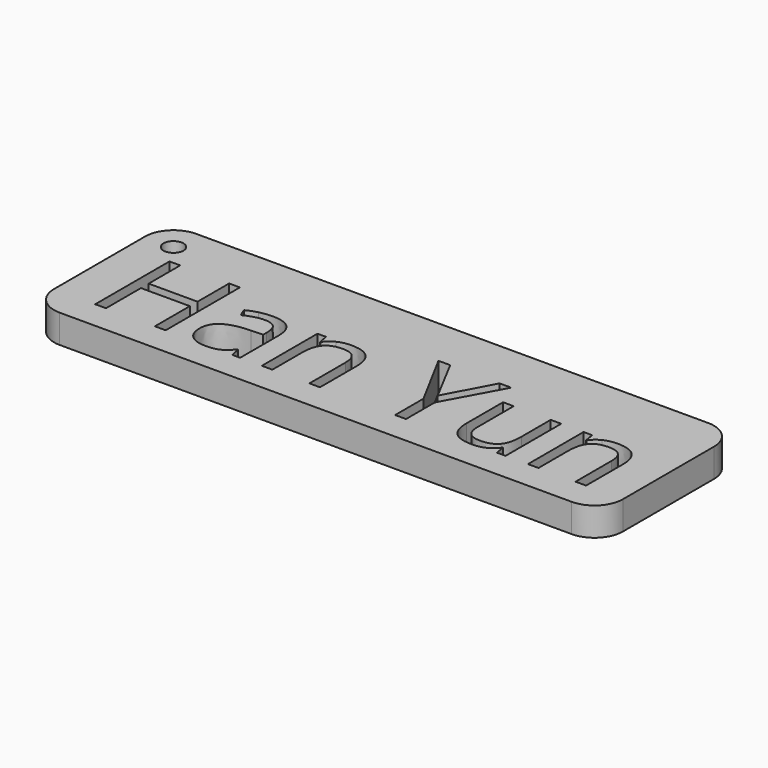
from build123d import *

# Parameters (mm, degrees)
F0_R     = 1.75
F1_DEPTH = 5


with BuildPart() as f1:
    # F0 (on Top) → F1 (new body)
    with BuildSketch(Plane.XY):
        with BuildLine():
            Line((95, 0), (5, 0))
            ThreePointArc((5, 0), (1.4644660941, -1.4644660941), (0, -5))
            Line((0, -5), (0, -25))
            ThreePointArc((0, -25), (1.4644660941, -28.5355339059), (5, -30))
            Line((5, -30), (95, -30))
            ThreePointArc((95, -30), (98.5355339059, -28.5355339059), (100, -25))
            Line((100, -25), (100, -5))
            ThreePointArc((100, -5), (98.5355339059, -1.4644660941), (95, 0))
        make_face()
        Polygon((19.6251784864, -8.6899095669), (19.6251784864, -25), (17.7296525464, -25), (17.7296525464, -17.3250832937), (9.137315564, -17.3250832937), (9.137315564, -25), (7.241789624, -25), (7.241789624, -8.6899095669), (9.137315564, -8.6899095669), (9.137315564, -15.6294621609), (17.7296525464, -15.6294621609), (17.7296525464, -8.6899095669), align=None, mode=Mode.SUBTRACT)
        with BuildLine():
            Line((32.7118039029, -25), (31.3374583532, -25))
            Line((31.3374583532, -25), (30.969776297, -23.2579723941))
            Line((30.969776297, -23.2579723941), (30.8805330795, -23.2579723941))
            add(Edge.make_bspline(
                [(30.8805330795, -23.2579723941), (29.9666825321, -24.4074250357), (29.0581865778, -24.8161589719)],
                knots=[0, 0, 0, 1, 1, 1], degree=2))
            add(Edge.make_bspline(
                [(29.0581865778, -24.8161589719), (28.1496906235, -25.2248929081), (26.7860542599, -25.2248929081)],
                knots=[0, 0, 0, 1, 1, 1], degree=2))
            add(Edge.make_bspline(
                [(26.7860542599, -25.2248929081), (24.9690623513, -25.2248929081), (23.9374107568, -24.2860542599)],
                knots=[0, 0, 0, 1, 1, 1], degree=2))
            add(Edge.make_bspline(
                [(23.9374107568, -24.2860542599), (22.9057591623, -23.3472156116), (22.9057591623, -21.6194669205)],
                knots=[0, 0, 0, 1, 1, 1], degree=2))
            add(Edge.make_bspline(
                [(22.9057591623, -21.6194669205), (22.9057591623, -17.917658258), (28.8279390766, -17.7391718229)],
                knots=[0, 0, 0, 1, 1, 1], degree=2))
            Line((28.8279390766, -17.7391718229), (30.9019514517, -17.6713469776))
            Line((30.9019514517, -17.6713469776), (30.9019514517, -16.9109947644))
            add(Edge.make_bspline(
                [(30.9019514517, -16.9109947644), (30.9019514517, -15.472394098), (30.2843883865, -14.7870061875)],
                knots=[0, 0, 0, 1, 1, 1], degree=2))
            add(Edge.make_bspline(
                [(30.2843883865, -14.7870061875), (29.6668253213, -14.101618277), (28.3031889576, -14.101618277)],
                knots=[0, 0, 0, 1, 1, 1], degree=2))
            add(Edge.make_bspline(
                [(28.3031889576, -14.101618277), (26.7753450738, -14.101618277), (24.8476915754, -15.0368871966)],
                knots=[0, 0, 0, 1, 1, 1], degree=2))
            Line((24.8476915754, -15.0368871966), (24.2765349833, -13.6197049024))
            add(Edge.make_bspline(
                [(24.2765349833, -13.6197049024), (25.1796763446, -13.1306520704), (26.2559495478, -12.8522132318)],
                knots=[0, 0, 0, 1, 1, 1], degree=2))
            add(Edge.make_bspline(
                [(26.2559495478, -12.8522132318), (27.3322227511, -12.5737743931), (28.4174202761, -12.5737743931)],
                knots=[0, 0, 0, 1, 1, 1], degree=2))
            add(Edge.make_bspline(
                [(28.4174202761, -12.5737743931), (30.6020942408, -12.5737743931), (31.6569490719, -13.5429557354)],
                knots=[0, 0, 0, 1, 1, 1], degree=2))
            add(Edge.make_bspline(
                [(31.6569490719, -13.5429557354), (32.7118039029, -14.5121370776), (32.7118039029, -16.653974298)],
                knots=[0, 0, 0, 1, 1, 1], degree=2))
            Line((32.7118039029, -16.653974298), (32.7118039029, -25))
        make_face(mode=Mode.SUBTRACT)
        with BuildLine():
            Line((46.744407425, -25), (44.8917182294, -25))
            Line((44.8917182294, -25), (44.8917182294, -17.0894811994))
            add(Edge.make_bspline(
                [(44.8917182294, -17.0894811994), (44.8917182294, -15.5973346026), (44.2116849119, -14.8601856259)],
                knots=[0, 0, 0, 1, 1, 1], degree=2))
            add(Edge.make_bspline(
                [(44.2116849119, -14.8601856259), (43.5316515945, -14.1230366492), (42.0787720133, -14.1230366492)],
                knots=[0, 0, 0, 1, 1, 1], degree=2))
            add(Edge.make_bspline(
                [(42.0787720133, -14.1230366492), (40.1618277011, -14.1230366492), (39.2693955259, -15.1600428367)],
                knots=[0, 0, 0, 1, 1, 1], degree=2))
            add(Edge.make_bspline(
                [(39.2693955259, -15.1600428367), (38.3769633508, -16.1970490243), (38.3769633508, -18.585197525)],
                knots=[0, 0, 0, 1, 1, 1], degree=2))
            Line((38.3769633508, -18.585197525), (38.3769633508, -25))
            Line((38.3769633508, -25), (36.5242741552, -25))
            Line((36.5242741552, -25), (36.5242741552, -12.7736792004))
            Line((36.5242741552, -12.7736792004), (38.0306996668, -12.7736792004))
            Line((38.0306996668, -12.7736792004), (38.3305568777, -14.447881961))
            Line((38.3305568777, -14.447881961), (38.4198000952, -14.447881961))
            add(Edge.make_bspline(
                [(38.4198000952, -14.447881961), (38.9909566873, -13.5447405997), (40.0172536887, -13.046763446)],
                knots=[0, 0, 0, 1, 1, 1], degree=2))
            add(Edge.make_bspline(
                [(40.0172536887, -13.046763446), (41.0435506901, -12.5487862922), (42.3036649215, -12.5487862922)],
                knots=[0, 0, 0, 1, 1, 1], degree=2))
            add(Edge.make_bspline(
                [(42.3036649215, -12.5487862922), (44.5133269871, -12.5487862922), (45.6288672061, -13.6143503094)],
                knots=[0, 0, 0, 1, 1, 1], degree=2))
            add(Edge.make_bspline(
                [(45.6288672061, -13.6143503094), (46.744407425, -14.6799143265), (46.744407425, -17.0252260828)],
                knots=[0, 0, 0, 1, 1, 1], degree=2))
            Line((46.744407425, -17.0252260828), (46.744407425, -25))
        make_face(mode=Mode.SUBTRACT)
        with BuildLine():
            Line((69.1444550214, -12.7736792004), (71.0185625892, -12.7736792004))
            Line((71.0185625892, -12.7736792004), (71.0185625892, -20.7056163732))
            add(Edge.make_bspline(
                [(71.0185625892, -20.7056163732), (71.0185625892, -22.2013326987), (71.6985959067, -22.936696811)],
                knots=[0, 0, 0, 1, 1, 1], degree=2))
            add(Edge.make_bspline(
                [(71.6985959067, -22.936696811), (72.3786292242, -23.6720609234), (73.8279390766, -23.6720609234)],
                knots=[0, 0, 0, 1, 1, 1], degree=2))
            add(Edge.make_bspline(
                [(73.8279390766, -23.6720609234), (75.7484531176, -23.6720609234), (76.6337458353, -22.6243455497)],
                knots=[0, 0, 0, 1, 1, 1], degree=2))
            add(Edge.make_bspline(
                [(76.6337458353, -22.6243455497), (77.5190385531, -21.5766301761), (77.5190385531, -19.1991908615)],
                knots=[0, 0, 0, 1, 1, 1], degree=2))
            Line((77.5190385531, -19.1991908615), (77.5190385531, -12.7736792004))
            Line((77.5190385531, -12.7736792004), (79.3717277487, -12.7736792004))
            Line((79.3717277487, -12.7736792004), (79.3717277487, -25))
            Line((79.3717277487, -25), (77.8438838648, -25))
            Line((77.8438838648, -25), (77.5761542123, -23.3614945264))
            Line((77.5761542123, -23.3614945264), (77.4762018087, -23.3614945264))
            add(Edge.make_bspline(
                [(77.4762018087, -23.3614945264), (76.9086149453, -24.2646358877), (75.898381723, -24.7447643979)],
                knots=[0, 0, 0, 1, 1, 1], degree=2))
            add(Edge.make_bspline(
                [(75.898381723, -24.7447643979), (74.8881485007, -25.2248929081), (73.5923369824, -25.2248929081)],
                knots=[0, 0, 0, 1, 1, 1], degree=2))
            add(Edge.make_bspline(
                [(73.5923369824, -25.2248929081), (71.3612565445, -25.2248929081), (70.252855783, -24.1646834841)],
                knots=[0, 0, 0, 1, 1, 1], degree=2))
            add(Edge.make_bspline(
                [(70.252855783, -24.1646834841), (69.1444550214, -23.10447406), (69.1444550214, -20.7734412185)],
                knots=[0, 0, 0, 1, 1, 1], degree=2))
            Line((69.1444550214, -20.7734412185), (69.1444550214, -12.7736792004))
        make_face(mode=Mode.SUBTRACT)
        Polygon((56.59328891, -8.6899095669), (60.9126606378, -16.8467396478), (65.2605901951, -8.6899095669), (67.313184198, -8.6899095669), (61.8693479296, -18.6744407425), (61.8693479296, -25), (59.9524036173, -25), (59.9524036173, -18.76368396), (54.519276535, -8.6899095669), align=None, mode=Mode.SUBTRACT)
        with BuildLine():
            Line((93.5185625892, -25), (91.6658733936, -25))
            Line((91.6658733936, -25), (91.6658733936, -17.0894811994))
            add(Edge.make_bspline(
                [(91.6658733936, -17.0894811994), (91.6658733936, -15.5973346026), (90.9858400762, -14.8601856259)],
                knots=[0, 0, 0, 1, 1, 1], degree=2))
            add(Edge.make_bspline(
                [(90.9858400762, -14.8601856259), (90.3058067587, -14.1230366492), (88.8529271775, -14.1230366492)],
                knots=[0, 0, 0, 1, 1, 1], degree=2))
            add(Edge.make_bspline(
                [(88.8529271775, -14.1230366492), (86.9359828653, -14.1230366492), (86.0435506901, -15.1600428367)],
                knots=[0, 0, 0, 1, 1, 1], degree=2))
            add(Edge.make_bspline(
                [(86.0435506901, -15.1600428367), (85.151118515, -16.1970490243), (85.151118515, -18.585197525)],
                knots=[0, 0, 0, 1, 1, 1], degree=2))
            Line((85.151118515, -18.585197525), (85.151118515, -25))
            Line((85.151118515, -25), (83.2984293194, -25))
            Line((83.2984293194, -25), (83.2984293194, -12.7736792004))
            Line((83.2984293194, -12.7736792004), (84.804854831, -12.7736792004))
            Line((84.804854831, -12.7736792004), (85.1047120419, -14.447881961))
            Line((85.1047120419, -14.447881961), (85.1939552594, -14.447881961))
            add(Edge.make_bspline(
                [(85.1939552594, -14.447881961), (85.7651118515, -13.5447405997), (86.7914088529, -13.046763446)],
                knots=[0, 0, 0, 1, 1, 1], degree=2))
            add(Edge.make_bspline(
                [(86.7914088529, -13.046763446), (87.8177058544, -12.5487862922), (89.0778200857, -12.5487862922)],
                knots=[0, 0, 0, 1, 1, 1], degree=2))
            add(Edge.make_bspline(
                [(89.0778200857, -12.5487862922), (91.2874821514, -12.5487862922), (92.4030223703, -13.6143503094)],
                knots=[0, 0, 0, 1, 1, 1], degree=2))
            add(Edge.make_bspline(
                [(92.4030223703, -13.6143503094), (93.5185625892, -14.6799143265), (93.5185625892, -17.0252260828)],
                knots=[0, 0, 0, 1, 1, 1], degree=2))
            Line((93.5185625892, -17.0252260828), (93.5185625892, -25))
        make_face(mode=Mode.SUBTRACT)
        with Locations((5, -5)):
            Circle(F0_R, mode=Mode.SUBTRACT)
    extrude(amount=F1_DEPTH)


solid = f1.part
